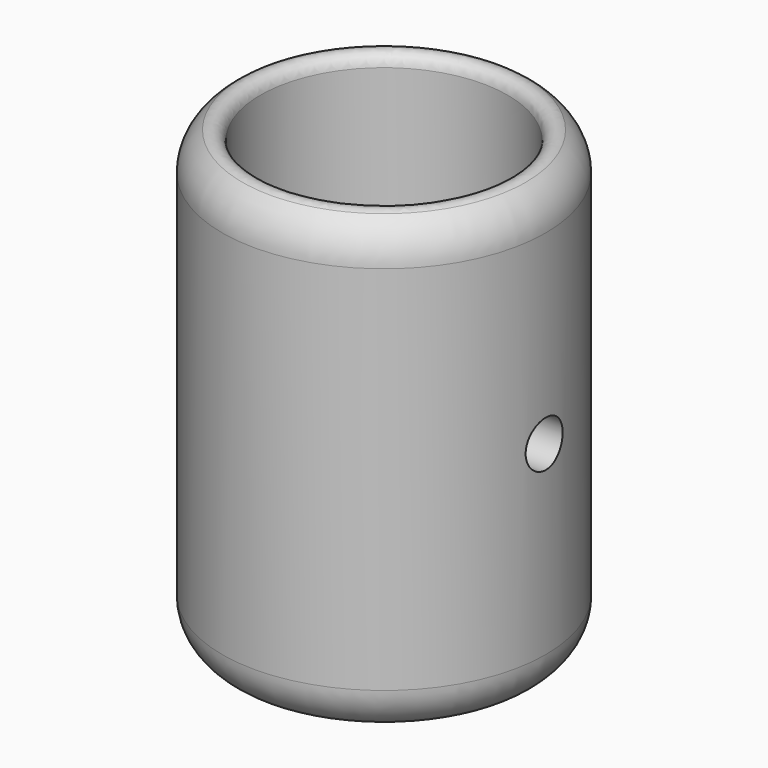
from build123d import *

# Parameters (mm, degrees)
F0_R     = 7
F0_R_2   = 5.35
F1_DEPTH = 20
F2_R     = 1
F3_DEPTH = 12.5
F5_R     = 0.5


# Not quite as in the source:
# - a fillet or chamfer that OpenCascade refuses, or shapes differently, is made with other operations: its cross-section is extruded or revolved along the edge and cut away or added


with BuildPart() as f1:
    # F0 (on Top) → F1 (new body)
    with BuildSketch(Plane.XY):
        Circle(F0_R)
        Circle(F0_R_2, mode=Mode.SUBTRACT)
    extrude(amount=F1_DEPTH)

    # F2 (on Right) → F3 (cut, symmetric)
    with BuildSketch(Plane.YZ):
        with Locations((0, 10)):
            Circle(F2_R)
    extrude(amount=F3_DEPTH, both=True, mode=Mode.SUBTRACT)

    # F4: fillet of radius 2 on 2 edges, made by hand

    # F4_s1 → F4_t2 (revolve, cut)
    with BuildSketch(Plane.XZ):
        with BuildLine():
            ThreePointArc((7, 18.0308631332), (6.5329709717, 19.3153863911), (5.35, 20))
            Line((5.35, 20), (7, 20))
            Line((7, 20), (7, 18.0308631332))
        make_face()
    revolve(axis=Axis((0, 0, 20), (0, 0, 1)), mode=Mode.SUBTRACT)

    # F4_s3 → F4_t4 (revolve, cut)
    with BuildSketch(Plane.XZ):
        with BuildLine():
            ThreePointArc((7, 1.9691368668), (6.5329709717, 0.6846136089), (5.35, 0))
            Line((5.35, 0), (7, 0))
            Line((7, 0), (7, 1.9691368668))
        make_face()
    revolve(axis=Axis((0, 0, 0), (0, 0, 1)), mode=Mode.SUBTRACT)

    # F5
    f5_edges = [f1.edges().sort_by_distance(p)[0] for p in [
        (-5.35, 0, 20),
        (-5.35, 0, 0),
    ]]
    fillet(f5_edges, radius=F5_R)


solid = f1.part
